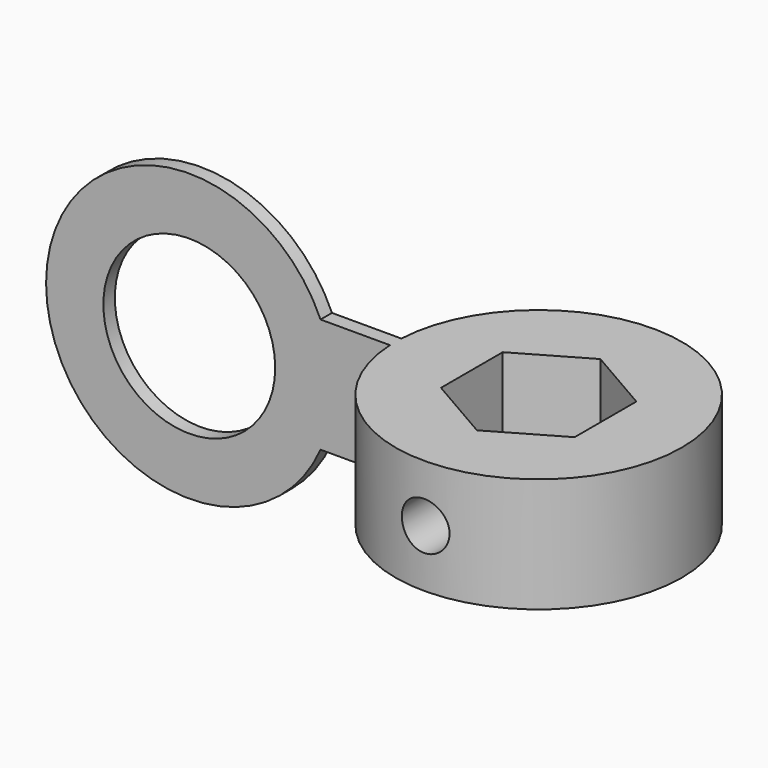
from build123d import *

# Parameters (mm, degrees)
F0_R      = 15
F1_DEPTH  = 12
F3_DEPTH  = 12.001
F4_R      = 15
F5_DEPTH  = 0.75
F6_R      = 9
F7_DEPTH  = 15.751
F9_R      = 2.5
F10_DEPTH = 12
F11_W     = 1.5
F11_H     = 12
F12_REACH = 42.0943866224
F13_W     = 1.5
F13_H     = 12
F14_DEPTH = 8


with BuildPart() as f1:
    # F0 (on Top) → F1 (new body)
    with BuildSketch(Plane.XY):
        Circle(F0_R)
    extrude(amount=F1_DEPTH)

    # F2 (on face) → F3 (cut, through all)
    with BuildSketch(Plane.XY.offset(12)):
        Polygon((7, -4.0414518843), (7, 4.0414518843), (0, 8.0829037687), (-7, 4.0414518843), (-7, -4.0414518843), (0, -8.0829037687), align=None)
    extrude(amount=-F3_DEPTH, mode=Mode.SUBTRACT)

    # F9 (on offset) → F10 (cut)
    with BuildSketch(Plane.XZ.offset(15)):
        with Locations((0, 6)):
            Circle(F9_R)
    extrude(amount=-F10_DEPTH, mode=Mode.SUBTRACT)



with BuildPart() as f5:
    # F4 (on Front) → F5 (new body, symmetric)
    with BuildSketch(Plane.XZ):
        with Locations((-36, 6)):
            Circle(F4_R)
    extrude(amount=F5_DEPTH, both=True)

    # F6 (on face) → F7 (cut, through all)
    with BuildSketch(Plane.XZ.offset(0.75)):
        with Locations((-36, 6)):
            Circle(F6_R)
    extrude(amount=-F7_DEPTH, mode=Mode.SUBTRACT)



with BuildPart() as f5b:
    # F4 (on Front) → F5, piece 2 (new body, symmetric)
    with BuildSketch(Plane.XZ):
        Polygon((-21, 0), (-15, 0), (-15, 12), (-21, 12), (-21, 6), align=None)
    extrude(amount=F5_DEPTH, both=True)


with BuildPart() as f5_1:
    add(f5.part)

    add(f5b.part)  # F12 merges F5b
    f12_end = f5_1.faces().sort_by_distance((-45, 0, 6))[0]
    # F11 (on face) → F12 (join, up to a face of the model that its end follows)
    with BuildSketch(Plane(origin=(-21, 0, 0), x_dir=(0, -1, 0), z_dir=(-1, 0, 0))):
        with Locations((0, 6)):
            Rectangle(F11_W, F11_H)
    f12_long = extrude(amount=F12_REACH, mode=Mode.PRIVATE)
    add(split(f12_long, bisect_by=f12_end, keep=Keep.ALL, mode=Mode.PRIVATE).solids().sort_by_distance((-21, 0, 6))[0])


with BuildPart() as f1_1:
    add(f1.part)

    add(f5_1.part)  # F14 merges F5
    # F13 (on face) → F14 (join, through all)
    with BuildSketch(Plane.YZ.offset(-15)):
        with Locations((0, 6)):
            Rectangle(F13_W, F13_H)
    extrude(amount=F14_DEPTH)


solid = f1_1.part
